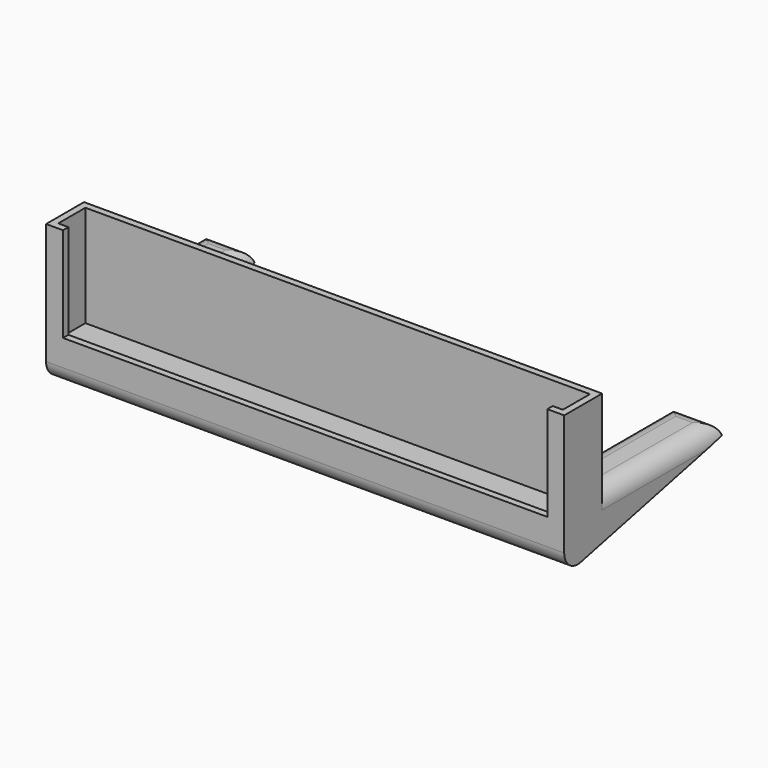
from build123d import *

# Parameters (mm, degrees)
F0_W         = 153
F0_H         = 14
F0_W_2       = 149
F0_H_2       = 10
F1_DEPTH     = 32
F2_DEPTH     = 2
F3_W         = 143
F3_H         = 28
F4_DEPTH     = 5
F5_DEPTH     = 10
F7_DEPTH     = 250
F8_DEPTH     = 153
F9_W         = 123
F9_H         = 17.8690971754
F10_DEPTH    = 125
F11_T1_DEPTH = 56.9422424436
F11_T3_DEPTH = 39.1070522291
F11_T5_DEPTH = 39.1070522291
F11_T7_DEPTH = 184.1889460466


# Not quite as in the source:
# - a fillet or chamfer that OpenCascade refuses, or shapes differently, is made with other operations: its cross-section is extruded or revolved along the edge and cut away or added


with BuildPart() as f1:
    # F0 (on Top) → F1 (new body)
    with BuildSketch(Plane.XY):
        with Locations((16.3109540343, 7)):
            Rectangle(F0_W, F0_H)
        with Locations((16.3109540343, 7)):
            Rectangle(F0_W_2, F0_H_2, mode=Mode.SUBTRACT)
    extrude(amount=F1_DEPTH)

    # F0 (on Top) → F2 (join)
    with BuildSketch(Plane.XY):
        with Locations((16.3109540343, 7)):
            Rectangle(F0_W_2, F0_H_2)
    extrude(amount=F2_DEPTH)

    # F3 (on face) → F4 (cut)
    with BuildSketch(Plane.XZ):
        with Locations((16.3109540343, 18)):
            Rectangle(F3_W, F3_H)
    extrude(amount=-F4_DEPTH, mode=Mode.SUBTRACT)

    # F0 (on Top) → F5 (join)
    with BuildSketch(Plane.XY):
        with Locations((16.3109540343, 7)):
            Rectangle(F0_W, F0_H)
        with Locations((16.3109540343, 7)):
            Rectangle(F0_W_2, F0_H_2, mode=Mode.SUBTRACT)
        with Locations((16.3109540343, 7)):
            Rectangle(F0_W_2, F0_H_2)
    extrude(amount=-F5_DEPTH)

    # F6 (on face) → F7 (cut)
    with BuildSketch(Plane(origin=(-60.1890459657, 0, 0), x_dir=(0, -1, 0), z_dir=(-1, 0, 0))):
        Polygon((-14, -10), (0, -10), (-14, -6.8780573927), align=None)
    extrude(amount=-F7_DEPTH, mode=Mode.SUBTRACT)

    # F6 (on face) → F8 (join)
    with BuildSketch(Plane(origin=(-60.1890459657, 0, 0), x_dir=(0, -1, 0), z_dir=(-1, 0, 0))):
        Polygon((-31.2427077442, -3.0330042519), (-14, -6.8780573927), (-14, 6.707993336), (-58.4422424436, 6.707993336), (-58.4422424436, 3.0323804822), align=None)
    extrude(amount=-F8_DEPTH)

    # F9 (on face) → F10 (cut)
    with BuildSketch(Plane(origin=(0, 14, 0), x_dir=(-1, 0, 0), z_dir=(0, 1, 0))):
        with Locations((-16.3109540343, -2.2265552517)):
            Rectangle(F9_W, F9_H)
    extrude(amount=F10_DEPTH, mode=Mode.SUBTRACT)

    # F11: fillet of radius 5 on 7 edges, made by hand

    # F11_s2 → F11_t1 (cut)
    with BuildSketch(Plane.XZ.offset(-70.9422424436)):
        with BuildLine():
            ThreePointArc((82.8109540343, 6.707993336), (79.2754201284, 5.243527242), (77.8109540343, 1.707993336))
            Line((77.8109540343, 1.707993336), (77.8109540343, 6.707993336))
            Line((77.8109540343, 6.707993336), (82.8109540343, 6.707993336))
        make_face()
        with BuildLine():
            ThreePointArc((92.8109540343, 1.707993336), (91.3464879403, 5.243527242), (87.8109540343, 6.707993336))
            Line((87.8109540343, 6.707993336), (92.8109540343, 6.707993336))
            Line((92.8109540343, 6.707993336), (92.8109540343, 1.707993336))
        make_face()
        with BuildLine():
            ThreePointArc((-50.1890459657, 6.707993336), (-46.6535120597, 5.243527242), (-45.1890459657, 1.707993336))
            Line((-45.1890459657, 1.707993336), (-45.1890459657, 6.707993336))
            Line((-45.1890459657, 6.707993336), (-50.1890459657, 6.707993336))
        make_face()
        with BuildLine():
            ThreePointArc((-55.1890459657, 6.707993336), (-58.7245798716, 5.243527242), (-60.1890459657, 1.707993336))
            Line((-60.1890459657, 1.707993336), (-60.1890459657, 6.707993336))
            Line((-60.1890459657, 6.707993336), (-55.1890459657, 6.707993336))
        make_face()
    extrude(amount=F11_T1_DEPTH, mode=Mode.SUBTRACT)

    # F11_s4 → F11_t3 (cut)
    with BuildSketch(Plane.YZ.offset(65.7574279198)):
        with BuildLine():
            ThreePointArc((53.6208319977, 6.707993336), (56.6521736371, 5.6842941125), (58.4422424436, 3.0323804822))
            Line((58.4422424436, 3.0323804822), (58.4422424436, 6.707993336))
            Line((58.4422424436, 6.707993336), (53.6208319977, 6.707993336))
        make_face()
    extrude(amount=F11_T3_DEPTH, mode=Mode.SUBTRACT)

    # F11_s6 → F11_t5 (cut)
    with BuildSketch(Plane.YZ.offset(-72.2425720802)):
        with BuildLine():
            ThreePointArc((53.6208319977, 6.707993336), (56.6521736371, 5.6842941125), (58.4422424436, 3.0323804822))
            Line((58.4422424436, 3.0323804822), (58.4422424436, 6.707993336))
            Line((58.4422424436, 6.707993336), (53.6208319977, 6.707993336))
        make_face()
    extrude(amount=F11_T5_DEPTH, mode=Mode.SUBTRACT)

    # F11_s8 → F11_t7 (cut)
    with BuildSketch(Plane.YZ.offset(-75.783518989)):
        with BuildLine():
            ThreePointArc((0, -3.7622107907), (1.8728007621, -7.663572723), (6.0882499707, -8.6423452152))
            Line((6.0882499707, -8.6423452152), (0, -10))
            Line((0, -10), (0, -3.7622107907))
        make_face()
    extrude(amount=F11_T7_DEPTH, mode=Mode.SUBTRACT)


solid = f1.part
